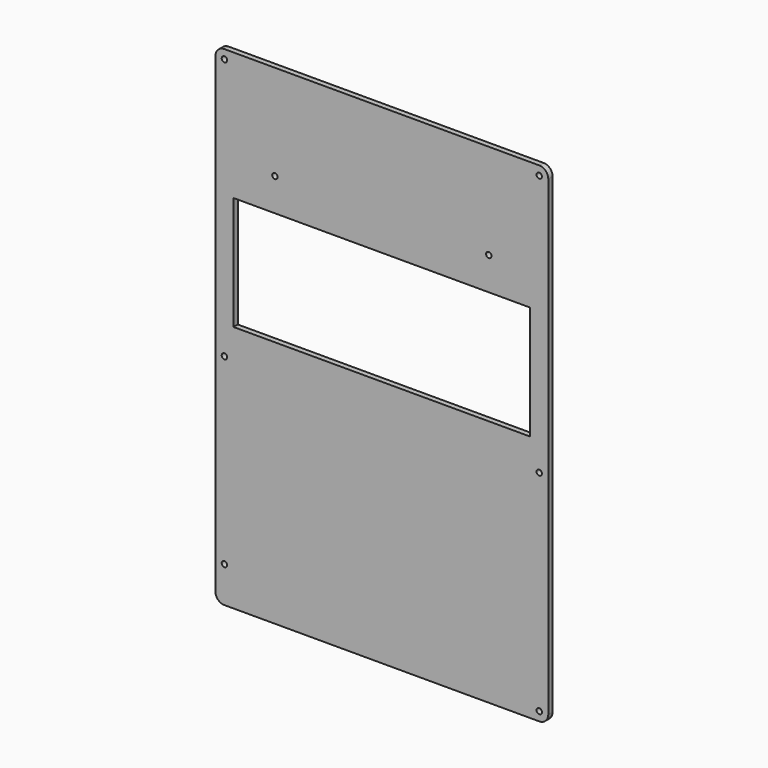
from build123d import *

# Parameters (mm, degrees)
F0_R     = 1.5
F0_W     = 40
F0_H     = 6.7
F0_H_2   = 1.6
F0_W_2   = 10
F0_H_3   = 91.46
F0_W_3   = 15
F0_H_4   = 1.7
F0_H_5   = 15
F0_H_6   = 5
F0_H_7   = 52.41
F0_H_8   = 3.65
F0_H_9   = 1.48
F0_W_4   = 3
F0_H_10  = 0.6
F0_H_11  = 1.4
F1_DEPTH = 2.9972


# Not quite as in the source:
# - a feature names something its author has since deleted; it is built from what else it names


with BuildPart() as f1:
    # F0 (on Front) → F1 (new body)
    with BuildSketch(Plane.XZ):
        with BuildLine():
            Line((-24.4680281997, 132.5136111658), (-91.7680281997, 132.5136111658))
            ThreePointArc((-91.7680281997, 132.5136111658), (-95.3035621056, 131.0491450717), (-96.7680281997, 127.5136111658))
            Line((-96.7680281997, 127.5136111658), (-96.7680281997, -22.4863888342))
            Line((-96.7680281997, -22.4863888342), (-86.7680281997, -22.4863888342))
            Line((-86.7680281997, -22.4863888342), (-86.7680281997, -1.5222273069))
            Line((-86.7680281997, -1.5222273069), (-86.7680281997, 0))
            Line((-86.7680281997, 0), (-86.7680281997, 16.1536111658))
            Line((-86.7680281997, 16.1536111658), (-86.7680281997, 20.4536111658))
            Line((-86.7680281997, 20.4536111658), (-86.7680281997, 21.4536111658))
            Line((-86.7680281997, 21.4536111658), (-89.7680281997, 21.4536111658))
            Line((-89.7680281997, 21.4536111658), (-89.7680281997, 22.0536111658))
            Line((-89.7680281997, 22.0536111658), (-89.7680281997, 22.8536111658))
            Line((-89.7680281997, 22.8536111658), (-89.7680281997, 23.4536111658))
            Line((-89.7680281997, 23.4536111658), (-86.7680281997, 23.4536111658))
            Line((-86.7680281997, 23.4536111658), (-86.7680281997, 24.4536111658))
            Line((-86.7680281997, 24.4536111658), (-86.7680281997, 24.6436111658))
            Line((-86.7680281997, 24.6436111658), (-86.7680281997, 53.4536111658))
            Line((-86.7680281997, 53.4536111658), (-86.7680281997, 56.4536111658))
            Line((-86.7680281997, 56.4536111658), (-86.7680281997, 60.7536111658))
            Line((-86.7680281997, 60.7536111658), (-86.7680281997, 61.4536111658))
            Line((-86.7680281997, 61.4536111658), (-86.7680281997, 122.5136111658))
            Line((-86.7680281997, 122.5136111658), (-40.4680281997, 122.5136111658))
            Line((-40.4680281997, 122.5136111658), (-39.4680281997, 122.5136111658))
            Line((-39.4680281997, 122.5136111658), (-39.4680281997, 124.2136111658))
            Line((-39.4680281997, 124.2136111658), (-49.4680281997, 124.2136111658))
            Line((-49.4680281997, 124.2136111658), (-49.4680281997, 125.8136111658))
            Line((-49.4680281997, 125.8136111658), (-28.7680281997, 125.8136111658))
            Line((-28.7680281997, 125.8136111658), (-24.4680281997, 125.8136111658))
            Line((-24.4680281997, 125.8136111658), (-24.4680281997, 132.5136111658))
        make_face()
        with Locations((-91.7680281997, -17.4863888342)):
            Circle(F0_R, mode=Mode.SUBTRACT)
        with Locations((-91.7680281997, 127.5136111658)):
            Circle(F0_R, mode=Mode.SUBTRACT)
        with Locations((-4.4680281997, 129.1636111658)):
            Rectangle(F0_W, F0_H)
        with BuildLine():
            Line((82.8319718003, 132.5136111658), (15.5319718003, 132.5136111658))
            Line((15.5319718003, 132.5136111658), (15.5319718003, 125.8136111658))
            Line((15.5319718003, 125.8136111658), (21.2319718003, 125.8136111658))
            Line((21.2319718003, 125.8136111658), (40.5319718003, 125.8136111658))
            Line((40.5319718003, 125.8136111658), (40.5319718003, 124.2136111658))
            Line((40.5319718003, 124.2136111658), (30.5319718003, 124.2136111658))
            Line((30.5319718003, 124.2136111658), (30.5319718003, 122.5136111658))
            Line((30.5319718003, 122.5136111658), (40.5319718003, 122.5136111658))
            Line((40.5319718003, 122.5136111658), (77.8319718003, 122.5136111658))
            Line((77.8319718003, 122.5136111658), (77.8319718003, 61.4536111658))
            Line((77.8319718003, 61.4536111658), (77.8319718003, 60.7536111658))
            Line((77.8319718003, 60.7536111658), (77.8319718003, 56.4536111658))
            Line((77.8319718003, 56.4536111658), (77.8319718003, 53.4536111658))
            Line((77.8319718003, 53.4536111658), (77.8319718003, 24.6436111658))
            Line((77.8319718003, 24.6436111658), (77.8319718003, 24.4536111658))
            Line((77.8319718003, 24.4536111658), (77.8319718003, 23.4536111658))
            Line((77.8319718003, 23.4536111658), (80.8319718003, 23.4536111658))
            Line((80.8319718003, 23.4536111658), (80.8319718003, 22.8536111658))
            Line((80.8319718003, 22.8536111658), (80.8319718003, 21.4536111658))
            Line((80.8319718003, 21.4536111658), (77.8319718003, 21.4536111658))
            Line((77.8319718003, 21.4536111658), (77.8319718003, 20.4536111658))
            Line((77.8319718003, 20.4536111658), (77.8319718003, 16.1536111658))
            Line((77.8319718003, 16.1536111658), (77.8319718003, 4.5))
            Line((77.8319718003, 4.5), (77.8319718003, -1.5222273069))
            Line((77.8319718003, -1.5222273069), (77.8319718003, -128.9463888342))
            Line((77.8319718003, -128.9463888342), (1.2319718003, -128.9463888342))
            Line((1.2319718003, -128.9463888342), (1.2319718003, -130.4263888342))
            Line((1.2319718003, -130.4263888342), (3.7319718003, -130.4263888342))
            Line((3.7319718003, -130.4263888342), (3.7319718003, -132.0263888342))
            Line((3.7319718003, -132.0263888342), (-11.2680281997, -132.0263888342))
            Line((-11.2680281997, -132.0263888342), (-11.2680281997, -130.4263888342))
            Line((-11.2680281997, -130.4263888342), (-8.7680281997, -130.4263888342))
            Line((-8.7680281997, -130.4263888342), (-8.7680281997, -128.9463888342))
            Line((-8.7680281997, -128.9463888342), (-86.7680281997, -128.9463888342))
            Line((-86.7680281997, -128.9463888342), (-96.7680281997, -128.9463888342))
            Line((-96.7680281997, -128.9463888342), (-96.7680281997, -132.2803888342))
            Line((-96.7680281997, -132.2803888342), (-96.7680281997, -133.9463888342))
            ThreePointArc((-96.7680281997, -133.9463888342), (-95.3035621056, -137.4819227401), (-91.7680281997, -138.9463888342))
            Line((-91.7680281997, -138.9463888342), (82.8319718003, -138.9463888342))
            ThreePointArc((82.8319718003, -138.9463888342), (86.3675057063, -137.4819227401), (87.8319718003, -133.9463888342))
            Line((87.8319718003, -133.9463888342), (87.8319718003, 127.5136111658))
            ThreePointArc((87.8319718003, 127.5136111658), (86.3675057063, 131.0491450717), (82.8319718003, 132.5136111658))
        make_face()
        with Locations((82.8319718003, -133.9463888342)):
            Circle(F0_R, mode=Mode.SUBTRACT)
        with Locations((82.8319718003, -17.4863888342)):
            Circle(F0_R, mode=Mode.SUBTRACT)
        with Locations((82.8319718003, 127.5136111658)):
            Circle(F0_R, mode=Mode.SUBTRACT)
        Polygon((-24.4680281997, 124.2136111658), (-24.4680281997, 125.8136111658), (-28.7680281997, 125.8136111658), (-49.4680281997, 125.8136111658), (-49.4680281997, 124.2136111658), (-39.4680281997, 124.2136111658), align=None)
        with Locations((-4.4680281997, 125.0136111658)):
            Rectangle(F0_W, F0_H_2)
        with Locations((-91.7680281997, -68.2163888342)):
            Rectangle(F0_W_2, F0_H_3)
        Polygon((21.2319718003, 125.8136111658), (15.5319718003, 125.8136111658), (15.5319718003, 124.2136111658), (30.5319718003, 124.2136111658), (40.5319718003, 124.2136111658), (40.5319718003, 125.8136111658), align=None)
        with Locations((-31.9680281997, 123.3636111658)):
            Rectangle(F0_W_3, F0_H_4)
        with Locations((-4.4680281997, 123.3636111658)):
            Rectangle(F0_W, F0_H_4)
        with Locations((-91.7680281997, -121.4463888342)):
            Rectangle(F0_W_2, F0_H_5)
        with Locations((-91.7680281997, -118.9463888342)):
            Circle(F0_R, mode=Mode.SUBTRACT)
        Polygon((-86.7680281997, -1.5222273069), (-86.7680281997, -22.4863888342), (-86.7680281997, -113.9463888342), (-86.7680281997, -128.9463888342), (-8.7680281997, -128.9463888342), (1.2319718003, -128.9463888342), (77.8319718003, -128.9463888342), (77.8319718003, -1.5222273069), align=None)
        with Locations((23.0319718003, 123.3636111658)):
            Rectangle(F0_W_3, F0_H_4)
        with Locations((-31.9680281997, 120.0136111658)):
            Rectangle(F0_W_3, F0_H_6)
        with Locations((-4.4680281997, 120.0136111658)):
            Rectangle(F0_W, F0_H_6)
        with Locations((23.0319718003, 120.0136111658)):
            Rectangle(F0_W_3, F0_H_6)
        Polygon((-39.4680281997, 117.5136111658), (-39.4680281997, 122.5136111658), (-40.4680281997, 122.5136111658), (-86.7680281997, 122.5136111658), (-86.7680281997, 61.4536111658), (-79.4680281997, 61.4536111658), (-79.4680281997, 65.1036111658), (-66.1611799171, 65.1036111658), align=None)
        with Locations((-63.7680281997, 79.6436111658)):
            Circle(F0_R, mode=Mode.SUBTRACT)
        Polygon((-24.4680281997, 65.1036111658), (-24.4680281997, 117.5136111658), (-39.4680281997, 117.5136111658), (-66.1611799171, 65.1036111658), align=None)
        with Locations((-4.4680281997, 91.3086111658)):
            Rectangle(F0_W, F0_H_7)
        Polygon((40.5319718003, 122.5136111658), (30.5319718003, 122.5136111658), (30.5319718003, 117.5136111658), (57.2251235178, 65.1036111658), (70.5319718003, 65.1036111658), (70.5319718003, 61.4536111658), (77.8319718003, 61.4536111658), (77.8319718003, 122.5136111658), align=None)
        with Locations((54.8319718003, 79.6436111658)):
            Circle(F0_R, mode=Mode.SUBTRACT)
        Polygon((30.5319718003, 117.5136111658), (15.5319718003, 117.5136111658), (15.5319718003, 65.1036111658), (57.2251235178, 65.1036111658), align=None)
        with Locations((-4.4680281997, 63.2786111658)):
            Rectangle(F0_W, F0_H_8)
        Polygon((-24.4680281997, 61.4536111658), (-24.4680281997, 65.1036111658), (-66.1611799171, 65.1036111658), (-68.0201763638, 61.4536111658), align=None)
        with Locations((-3.7680281997, -129.6863888342)):
            Rectangle(F0_W_2, F0_H_9)
        Polygon((57.2251235178, 65.1036111658), (15.5319718003, 65.1036111658), (15.5319718003, 61.4536111658), (59.0841199644, 61.4536111658), align=None)
        Polygon((-68.0201763638, 61.4536111658), (-66.1611799171, 65.1036111658), (-79.4680281997, 65.1036111658), (-79.4680281997, 61.4536111658), align=None)
        Polygon((1.2319718003, -130.4263888342), (-8.7680281997, -130.4263888342), (-11.2680281997, -130.4263888342), (-11.2680281997, -132.0263888342), (3.7319718003, -132.0263888342), (3.7319718003, -130.4263888342), align=None)
        Polygon((70.5319718003, 65.1036111658), (57.2251235178, 65.1036111658), (59.0841199644, 61.4536111658), (70.5319718003, 61.4536111658), align=None)
        Polygon((-89.7680281997, 21.4536111658), (-86.7680281997, 21.4536111658), (-86.7680281997, 22.8536111658), (-89.7680281997, 22.8536111658), (-89.7680281997, 22.0536111658), align=None)
        with Locations((-88.2680281997, 23.1536111658)):
            Rectangle(F0_W_4, F0_H_10)
        with Locations((79.3319718003, 22.1536111658)):
            Rectangle(F0_W_4, F0_H_11)
        with Locations((79.3319718003, 23.1536111658)):
            Rectangle(F0_W_4, F0_H_10)
    extrude(amount=F1_DEPTH)


solid = f1.part
